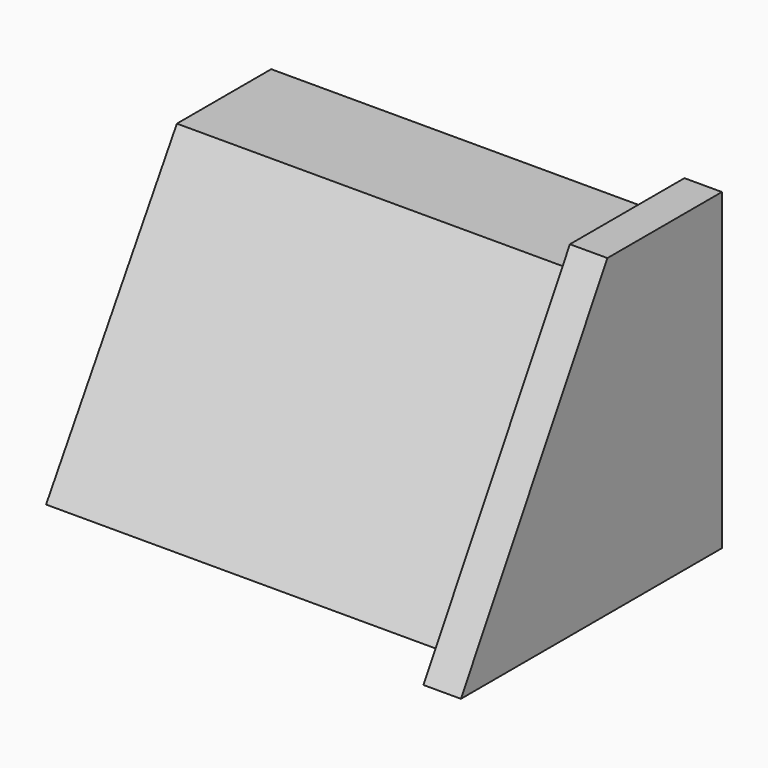
from build123d import *

# Parameters (mm, degrees)
F0_W     = 119.6608580649
F0_H     = 94.0911695361
F1_DEPTH = 79.502
F3_DEPTH = 92.71
F5_DEPTH = 135.4624384472
F7_DEPTH = 11.086793376


with BuildPart() as f1:
    # F0 (on Top) → F1 (new body)
    with BuildSketch(Plane.XY):
        with Locations((-1.6834978014, -1.9669607282)):
            Rectangle(F0_W, F0_H)
    extrude(amount=F1_DEPTH)

    # F4 (on face) → F5 (cut, through all)
    with BuildSketch(Plane(origin=(-61.5139268339, 0, 0), x_dir=(0, -1, 0), z_dir=(-1, 0, 0))):
        Polygon((-10.2190570906, 79.502), (38.1188131869, 0), (49.0125454962, 0), (49.0125454962, 5.3254961967), (49.0125454962, 79.502), align=None)
    extrude(amount=-F5_DEPTH, mode=Mode.SUBTRACT)


with BuildPart() as f3:
    # F2 (on Top) → F3 (new body)
    with BuildSketch(Plane.XY):
        Polygon((73.9475116134, 42.3180349171), (62.8617182374, 42.3180349171), (62.8617182374, -52.922450006), (62.8617182374, -60.81943959), (73.9475116134, -60.81943959), align=None)
    extrude(amount=F3_DEPTH)

    # F6 (on face) → F7 (cut, through all)
    with BuildSketch(Plane(origin=(62.8617182374, 0, 0), x_dir=(0, -1, 0), z_dir=(-1, 0, 0))):
        Polygon((0, 92.71), (54.1358701885, 0), (60.81943959, 0), (60.81943959, 92.71), align=None)
    extrude(amount=-F7_DEPTH, mode=Mode.SUBTRACT)


solid = Compound([f1.part, f3.part])
